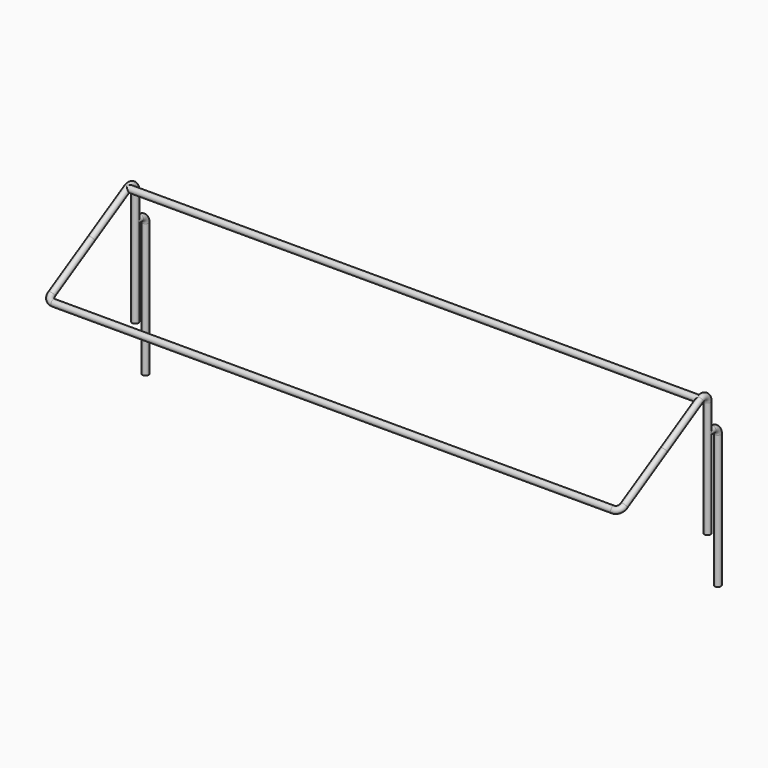
from build123d import *

# Parameters (mm, degrees)
F9_R  = 2.5
F8_R  = 2.5
F14_R = 2.5
F11_R = 2.5


with BuildPart() as f12:
    # F12: sweep along a path in F3, F5, F4
    with BuildLine(Plane.YZ) as f12_path:
        Line((0, -100), (0, -8.6602540378))
        ThreePointArc((0, -8.6602540378), (-2.5, -4.3301270189), (-7.5, -4.3301270189))
        Line((-7.5, -4.3301270189), (-43.3012701892, -25))
    with BuildLine(Plane(origin=(0, 0, 0), x_dir=(1, 0, 0), z_dir=(0, -0.5, 0.8660254038))) as f12_path_2:
        Line((0, -50), (0, -95))
        ThreePointArc((0, -95), (-1.4644660941, -98.5355339059), (-5, -100))
        Line((-5, -100), (-445, -100))
        ThreePointArc((-445, -100), (-448.5355339059, -98.5355339059), (-450, -95))
        Line((-450, -95), (-450, -50))
    with BuildLine(Plane.YZ.offset(-450)) as f12_path_3:
        Line((-43.3012701892, -25), (-7.5, -4.3301270189))
        ThreePointArc((-7.5, -4.3301270189), (-2.5, -4.3301270189), (0, -8.6602540378))
        Line((0, -8.6602540378), (0, -100))
    # F9 (on plane+point) → F12 (sweep)
    with BuildSketch(Plane.XY.offset(-100)):
        Circle(F9_R)
    sweep(path=f12_path.line + f12_path_2.line + f12_path_3.line)

    # F13: sweep along a path in F3
    with BuildLine(Plane.YZ) as f13_path:
        Line((10, -140), (10, -35))
        ThreePointArc((10, -35), (8.5355339059, -31.4644660941), (5, -30))
        Line((5, -30), (0, -30))
    # F8 (on plane+point) → F13 (sweep)
    with BuildSketch(Plane.XY.offset(-140)):
        with Locations((0, 10)):
            Circle(F8_R)
    sweep(path=f13_path.line)

    # F15: sweep along a path in F4
    with BuildLine(Plane.YZ.offset(-450)) as f15_path:
        Line((10, -140), (10, -35))
        ThreePointArc((10, -35), (8.5355339059, -31.4644660941), (5, -30))
        Line((5, -30), (0, -30))
    # F14 (on plane+point) → F15 (sweep)
    with BuildSketch(Plane.XY.offset(-140)):
        with Locations((-450, 10)):
            Circle(F14_R)
    sweep(path=f15_path.line)

    # F16: sweep along a path in F5
    with BuildLine(Plane(origin=(0, 0, 0), x_dir=(1, 0, 0), z_dir=(0, -0.5, 0.8660254038))) as f16_path:
        Line((-450, -8.6602540378), (0, -8.6602540378))
    # F11 (on offset) → F16 (sweep)
    with BuildSketch(Plane.YZ.offset(-25)):
        with Locations((-7.5, -4.3301270189)):
            Circle(F11_R)
    sweep(path=f16_path.line)


solid = f12.part
